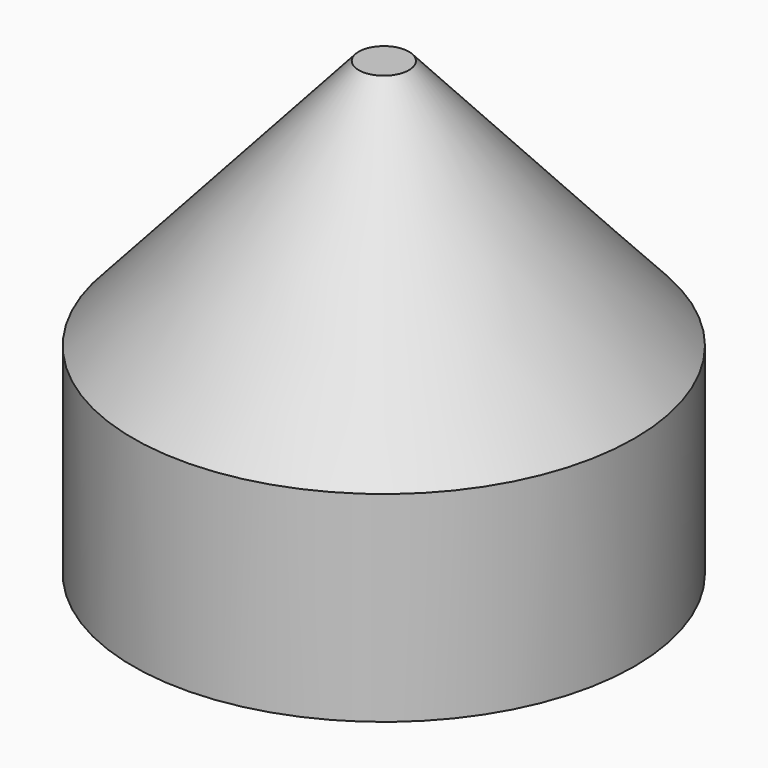
from build123d import *

# Parameters (mm, degrees)
F0_R           = 10
F0_R_2         = 6.1
F1_DEPTH       = 6
F2_DEPTH       = 10
F4_R           = 1
F1_FACE_R      = 10
F7_D           = 4.2
F7_CBORE_D     = 7
F7_CBORE_DEPTH = 4
F8_D           = 3.2
F8_DEPTH       = 8
F8_START       = 6
F8_TIP         = 0.9613769904
F6_R           = 10
F10_DEPTH      = 8
F12_DEPTH      = 10


with BuildPart() as f1:
    # F0 (on Top) → F1 (new body)
    with BuildSketch(Plane.XY):
        Circle(F0_R)
        Circle(F0_R_2, mode=Mode.SUBTRACT)
        Circle(F0_R_2)
    extrude(amount=F1_DEPTH)

    # F0 (on Top) → F2 (join)
    with BuildSketch(Plane.XY):
        Circle(F0_R)
        Circle(F0_R_2, mode=Mode.SUBTRACT)
    extrude(amount=-F2_DEPTH)

    # F7 (through all)
    with Locations(Plane(origin=(0, 0, 0), x_dir=(1, 0, 0), z_dir=(0, 0, -1))):
        with Locations((0, 0)):
            CounterBoreHole(F7_D / 2, F7_CBORE_D / 2, F7_CBORE_DEPTH)


with BuildPart() as f5:
    # F4 (on offset) → F5 section 0
    with BuildSketch(Plane.XY.offset(16)):
        Circle(F4_R)
    # F1_face (on face) → F5 section 1
    with BuildSketch(Plane.XY.offset(6)):
        Circle(F1_FACE_R)
    loft()

    # F8
    # its depths count from where the whole tool has entered the part; down to there all is cleared
    with Locations(Plane(origin=(0, 0, 0), x_dir=(1, 0, 0), z_dir=(0, 0, -1)).offset(-F8_START)):
        with Locations((0, 0)):
            Hole(F8_D / 2, depth=F8_DEPTH)
            with Locations((0, 0, -(F8_DEPTH + F8_TIP / 2))):  # 118° drill point
                Cone(0, F8_D / 2, F8_TIP, mode=Mode.SUBTRACT)

    # F6 (on face) → F10 (join)
    with BuildSketch(Plane.XY.offset(6)):
        Circle(F6_R)
    extrude(amount=-F10_DEPTH)

    # F11 (on face) → F12 (cut)
    with BuildSketch(Plane(origin=(0, 0, -2), x_dir=(1, 0, 0), z_dir=(0, 0, -1))):
        with BuildLine():
            ThreePointArc((1.6, 0), (0, 1.6), (-1.6, 0))
            ThreePointArc((-1.6, 0), (0, -1.6), (1.6, 0))
        make_face()
    extrude(amount=-F12_DEPTH, mode=Mode.SUBTRACT)


solid = f5.part
